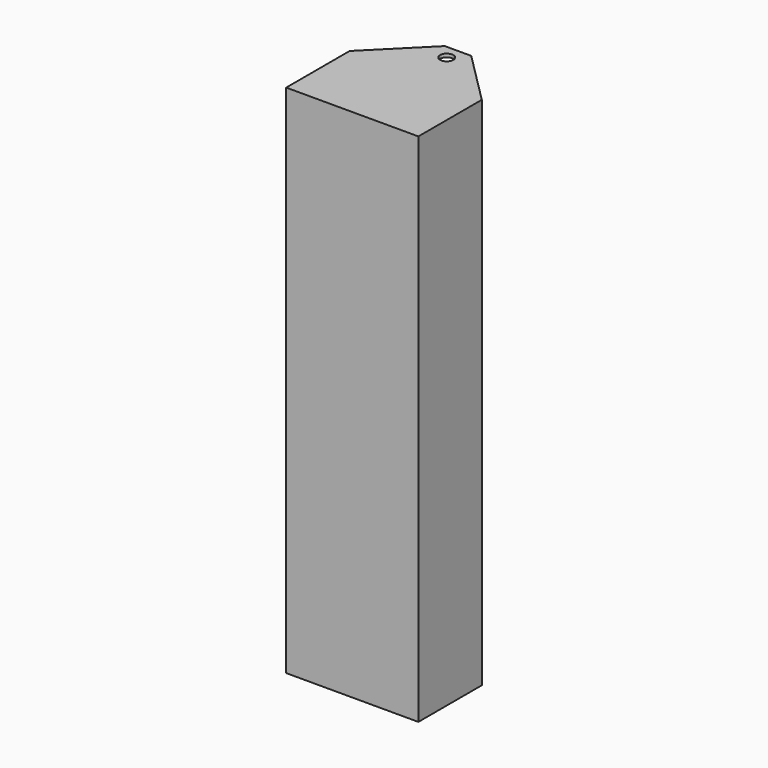
from build123d import *

# Parameters (mm, degrees)
F0_W        = 100
F0_H        = 100
F1_DEPTH    = 390
F2_T        = -2.5
F3_R        = 5
F4_DEPTH    = 2000
F5_T1_DEPTH = 595.7346390373
F6_W        = 95
F6_H        = 2.5
F7_DEPTH    = 59.6


# Not quite as in the source:
# - a fillet or chamfer that OpenCascade refuses, or shapes differently, is made with other operations: its cross-section is extruded or revolved along the edge and cut away or added


with BuildPart() as f1:
    # F0 (on Top) → F1 (new body)
    with BuildSketch(Plane.XY):
        with Locations((50, 50)):
            Rectangle(F0_W, F0_H)
    extrude(amount=F1_DEPTH)

    # F2
    f2_openings = [f1.faces().sort_by_distance(p)[0] for p in [
        (50, 100, 195),
    ]]
    offset(amount=F2_T, openings=f2_openings)

    # F3 (on face) → F4 (cut)
    with BuildSketch(Plane(origin=(0, 0, 0), x_dir=(1, 0, 0), z_dir=(0, 0, -1))):
        with Locations((50, -89.3280655146)):
            Circle(F3_R)
    extrude(amount=-F4_DEPTH, mode=Mode.SUBTRACT)

    # F5: chamfer of 40 on 2 edges, made by hand

    # F5_s2 → F5_t1 (cut)
    with BuildSketch(Plane.XY.offset(-102.8673195186)):
        Polygon((0, 60), (40, 100), (0, 100), align=None)
        Polygon((60, 100), (100, 60), (100, 100), align=None)
    extrude(amount=F5_T1_DEPTH, mode=Mode.SUBTRACT)

    # F6 (on face) → F7 (join)
    with BuildSketch(Plane(origin=(0, 2.5, 0), x_dir=(-1, 0, 0), z_dir=(0, 1, 0))):
        with Locations((-50, 328.2103848457)):
            Rectangle(F6_W, F6_H)
        with Locations((-50, 257.6169383526)):
            Rectangle(F6_W, F6_H)
        with Locations((-50, 151.1440885067)):
            Rectangle(F6_W, F6_H)
    extrude(amount=F7_DEPTH)


solid = f1.part
